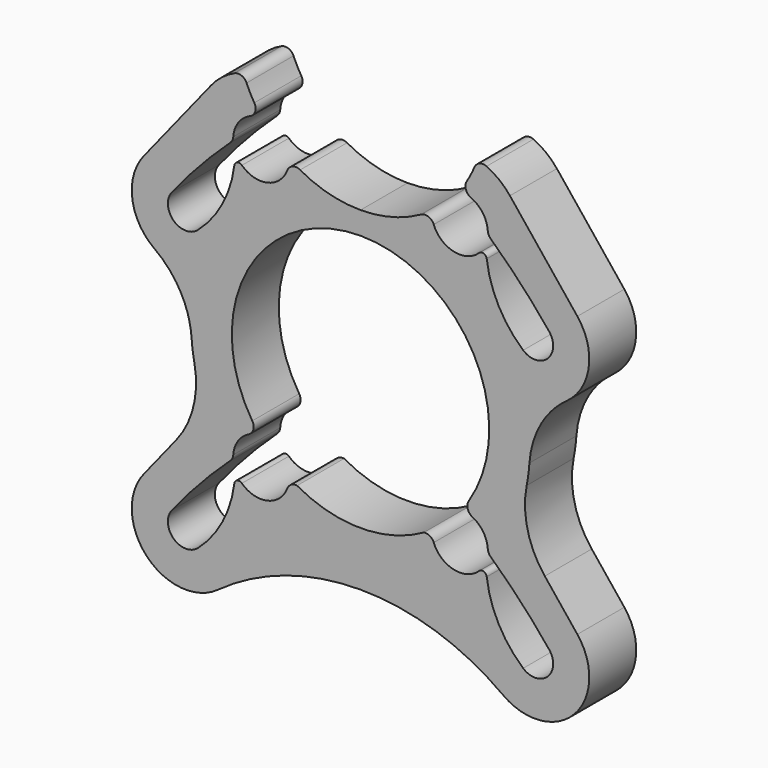
from build123d import *

# Parameters (mm, degrees)
F2_DEPTH       = 1.625
F3_R           = 0.5
F4_R           = 0.25
F9_DEPTH       = 1.625
F10_R          = 5
F11_R          = 7.125
F12_DEPTH      = 1.6260001
F12_DEPTH_BACK = 1.6260001
F13_R          = 0.5


# Not quite as in the source:
# - two fillets or chamfers of one size are made in one step
# - a feature names something its author has since deleted; it is built from what else it names


with BuildPart() as f2:
    # F1 (on Front) → F2 (new body, symmetric)
    with BuildSketch(Plane.XZ):
        with BuildLine():
            ThreePointArc((0, -6.875), (-2.0724417463, -6.5551971906), (-3.9520768911, -5.6255411515))
            ThreePointArc((-3.9520768911, -5.6255411515), (-4.8570002775, -7.1160909953), (-6.5757097792, -6.8217054979))
            ThreePointArc((-6.5757097792, -6.8217054979), (-6.7881621448, -6.5678083652), (-6.9418497803, -6.2745851185))
            ThreePointArc((-6.9418497803, -6.2745851185), (-7.4898612723, -8.7489164009), (-9.0066893746, -10.7791539234))
            ThreePointArc((-9.0066893746, -10.7791539234), (-10.3561219729, -10.7473840389), (-10.4445927673, -9.400479966))
            ThreePointArc((-10.4445927673, -9.400479966), (-8.8177667586, -7.5260240462), (-7.0479231089, -5.7859661986))
            ThreePointArc((-7.0479231089, -5.7859661986), (-6.6159518229, -4.6300438958), (-5.4766665535, -4.1559293139))
            ThreePointArc((-5.4766665535, -4.1559293139), (-6.0508763421, -3.2638199234), (-6.4809915278, -2.2939864464))
            ThreePointArc((-6.4809915278, -2.2939864464), (-7.4684871278, -2.7515095369), (-8.2709699391, -3.4866940551))
            Line((-8.2709699391, -3.4866940551), (-12.0057025921, -8.1503055323))
            ThreePointArc((-12.0057025921, -8.1503055323), (-11.8324993376, -12.098674705), (-7.8959026306, -12.4491384793))
            ThreePointArc((-7.8959026306, -12.4491384793), (-4.1524531082, -10.534781214), (0, -9.875))
            Line((0, -9.875), (0, -6.875))
        make_face()
    extrude(amount=F2_DEPTH, both=True)

    # F3
    f3_edges = [f2.edges().sort_by_distance(p)[0] for p in [
        (-3.952077, 0, -5.625541),
        (-7.047923, 0, -5.785966),
        (-6.480992, 0, -2.293986),
    ]]
    fillet(f3_edges, radius=F3_R)

    # F4
    f4_edges = [f2.edges().sort_by_distance(p)[0] for p in [
        (-6.94185, 0, -6.274585),
    ]]
    fillet(f4_edges, radius=F4_R)

    # F5: F2 across plane


with BuildPart() as f2_1:
    add(f2.part)
    add(f2.part.mirror(Plane.YZ))


with BuildPart() as f7_1:
    # F7: copy of F2
    add(f2_1.part.moved(Location((0, 0, 15.5))))


with BuildPart() as f2_2:
    add(f2_1.part)

    add(f7_1.part)  # F9 merges F7_1
    # F8 (on Front) → F9 (join, symmetric)
    with BuildSketch(Plane.XZ):
        with BuildLine():
            ThreePointArc((4.4191648166, 5.2665555464), (6.770553302, 1.1938312215), (5.953924651, -3.4375))
            Line((5.953924651, -3.4375), (8.1189881605, -4.6875))
            ThreePointArc((8.1189881605, -4.6875), (9.2325726845, 1.6279516656), (6.0261338408, 7.1816666542))
            Line((6.0261338408, 7.1816666542), (4.4191648166, 5.2665555464))
        make_face()
        with BuildLine():
            ThreePointArc((-6.0261338408, 7.1816666542), (-9.2325726845, 1.6279516656), (-8.1189881605, -4.6875))
            Line((-8.1189881605, -4.6875), (-5.953924651, -3.4375))
            ThreePointArc((-5.953924651, -3.4375), (-6.770553302, 1.1938312215), (-4.4191648166, 5.2665555464))
            Line((-4.4191648166, 5.2665555464), (-6.0261338408, 7.1816666542))
        make_face()
    extrude(amount=F9_DEPTH, both=True)

    # F10
    f10_edges = [f2_2.edges().sort_by_distance(p)[0] for p in [
        (8.552996, 0, -3.838864),
        (9.023329, 0, 2.543649),
        (-9.023329, 0, 2.543649),
        (-8.552996, 0, -3.838864),
    ]]
    fillet(f10_edges, radius=F10_R)

    # F11 (on Front) → F12 (cut, two sides)
    with BuildSketch(Plane.XZ) as f12_sk:
        with Locations((0, 0.25)):
            Circle(F11_R)
    extrude(amount=-F12_DEPTH, mode=Mode.SUBTRACT)
    extrude(f12_sk.sketch, amount=F12_DEPTH_BACK, mode=Mode.SUBTRACT)

    # F13
    f13_edges = [f2_2.edges().sort_by_distance(p)[0] for p in [
        (-5.597151, 0, -4.158801),
        (5.597151, 0, -4.158801),
        (-5.476667, 0, 11.344071),
        (5.476667, 0, 11.344071),
    ]]
    fillet(f13_edges, radius=F13_R)


solid = f2_2.part
